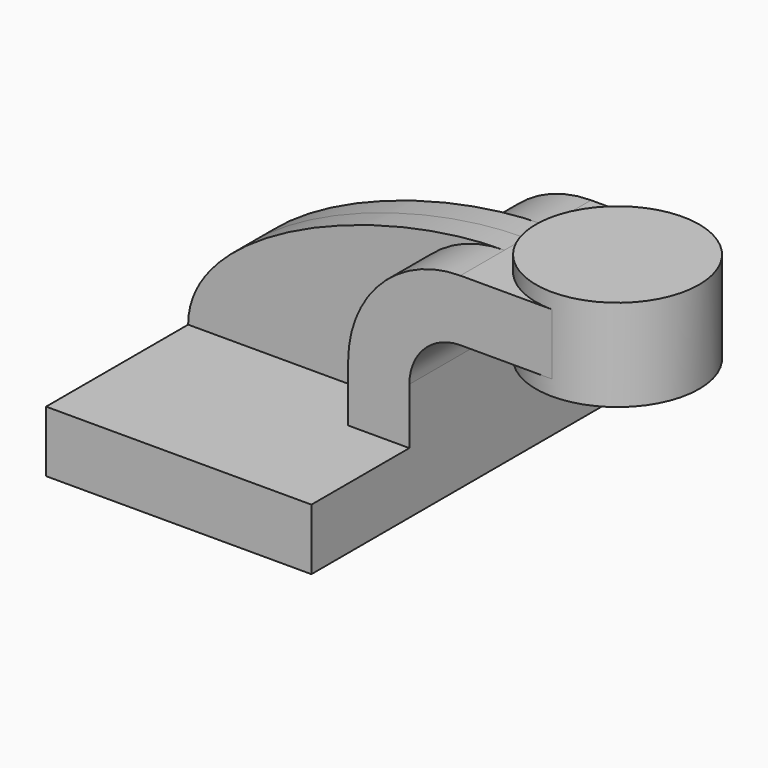
from build123d import *

# Parameters (mm, degrees)
F1_DEPTH = 63.5
F0_W     = 25.4
F0_H     = 19.05
F2_DEPTH = 25.4
F3_DEPTH = 8.255


with BuildPart() as f1:
    # F0 (on Front) → F1 (new body, symmetric)
    with BuildSketch(Plane.XZ):
        Polygon((41.275, -9.525), (41.275, 9.525), (22.225, 9.525), (-41.275, 9.525), (-41.275, -9.525), align=None)
    extrude(amount=F1_DEPTH, both=True)

    # F0 (on Front) → F2 (join, symmetric)
    with BuildSketch(Plane.XZ):
        with BuildLine():
            Line((22.225, 9.525), (41.275, 9.525))
            Line((41.275, 9.525), (41.275, 27.0002))
            ThreePointArc((41.275, 27.0002), (45.9246798487, 38.2255201513), (57.15, 42.8752))
            Line((57.15, 42.8752), (60.325, 42.8752))
            Line((60.325, 42.8752), (60.325, 61.9252))
            Line((60.325, 61.9252), (57.15, 61.9252))
            ThreePointArc((57.15, 61.9252), (32.4542956671, 51.6959043329), (22.225, 27.0002))
            Line((22.225, 27.0002), (22.225, 9.525))
        make_face()
        with Locations((73.025, 52.4002)):
            Rectangle(F0_W, F0_H)
    extrude(amount=F2_DEPTH, both=True)

    # F0 (on Front) → F3 (join, symmetric)
    with BuildSketch(Plane.XZ):
        with BuildLine():
            Line((-41.275, 9.525), (22.225, 9.525))
            Line((22.225, 9.525), (22.225, 27.0002))
            ThreePointArc((22.225, 27.0002), (32.4542956671, 51.6959043329), (57.15, 61.9252))
            add(Edge.make_bspline(
                [(-41.275, 9.525), (-41.275, 38.1), (16.719141975, 61.9252), (57.15, 61.9252)],
                knots=[0, 0, 0, 0, 111.5045361635, 111.5045361635, 111.5045361635, 111.5045361635], degree=3))
        make_face()
    extrude(amount=F3_DEPTH, both=True)

    # F0 (on Front) → F4 (revolve)
    with BuildSketch(Plane.XZ):
        Polygon((85.725, 61.9252), (85.725, 42.8752), (85.725, 38.1), (111.125, 38.1), (111.125, 66.675), (85.725, 66.675), align=None)
    revolve(axis=Axis((85.725, 0, 52.3875), (0, 0, 1)))


solid = f1.part
